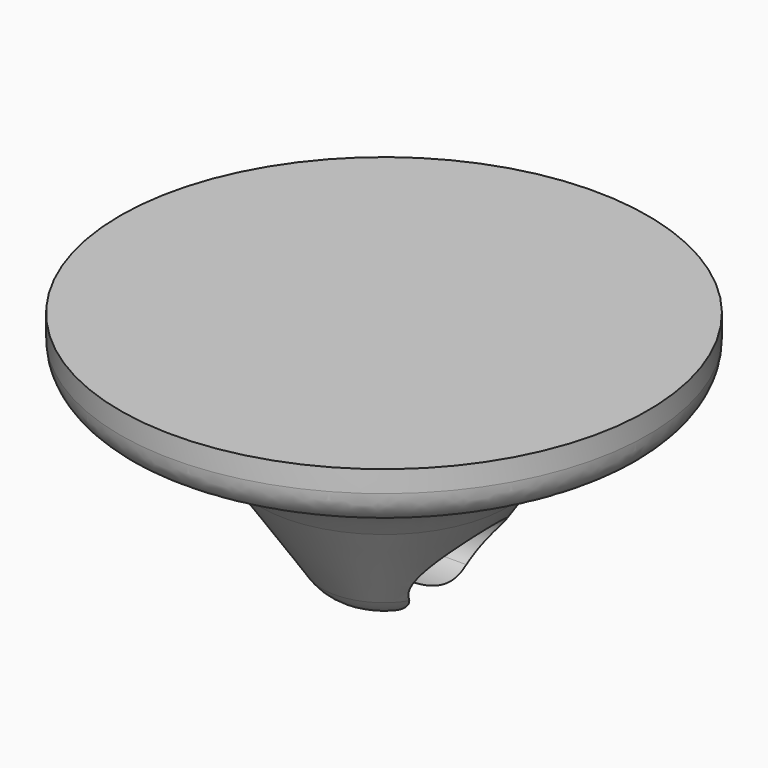
from build123d import *

# Parameters (mm, degrees)
F3_R          = 2
F4_R          = 3
F6_DEPTH      = 15.0010001
F6_DEPTH_BACK = 15.0010001
F7_T1_DEPTH   = 11.5921148274


# Not quite as in the source:
# - a fillet or chamfer that OpenCascade refuses, or shapes differently, is made with other operations: its cross-section is extruded or revolved along the edge and cut away or added
# - a feature of the source that left no trace in its solid (it failed there, or was rolled back) is left out


with BuildPart() as f1:
    # F0 (on Front) → F1 (revolve)
    with BuildSketch(Plane.XZ):
        Polygon((0, -13.9897428453), (0, 0), (-15, 0), (-15, -3), (-10, -3), (-2.61932757, -13.9897428453), align=None)
    revolve(axis=Axis((0, 0, -6.9948714226), (0, 0, 1)))

    # F2: fillet of radius 10 on 1 edges, made by hand

    # F2_s1 → F2_t2 (revolve)
    with BuildSketch(Plane.XZ):
        with BuildLine():
            ThreePointArc((-15, -3), (-10.4835294041, -4.2493813133), (-7.0321290602, -7.4191283024))
            Line((-7.0321290602, -7.4191283024), (-10, -3))
            Line((-10, -3), (-15, -3))
        make_face()
    revolve(axis=Axis((0, 0, -3), (0, 0, 1)))

    # F3
    f3_edges = [f1.edges().sort_by_distance(p)[0] for p in [
        (15, 0, -3),
    ]]
    fillet(f3_edges, radius=F3_R)

    # F4
    f4_edges = [f1.edges().sort_by_distance(p)[0] for p in [
        (2.619328, 0, -13.989743),
    ]]
    fillet(f4_edges, radius=F4_R)

    # F5 (on Right) → F6 (cut, two sides)
    with BuildSketch(Plane.YZ) as f6_sk:
        with BuildLine():
            Line((1.5, -14.6206104997), (1.5, -12.9897428453))
            ThreePointArc((1.5, -12.9897428453), (0, -8.4897428453), (-1.5, -12.9897428453))
            Line((-1.5, -12.9897428453), (-1.5, -14.6206104997))
            Line((-1.5, -14.6206104997), (1.5, -14.6206104997))
        make_face()
    extrude(amount=-F6_DEPTH, mode=Mode.SUBTRACT)
    extrude(f6_sk.sketch, amount=F6_DEPTH_BACK, mode=Mode.SUBTRACT)

    # F7: fillet of radius 3 on 2 edges, made by hand

    # F7_s2 → F7_t1 (cut)
    with BuildSketch(Plane.YZ.offset(-5.7960574137)):
        with BuildLine():
            ThreePointArc((-2.0454545455, -12.4271417817), (-1.6396122323, -13.2474864717), (-1.5, -14.1520205055))
            Line((-1.5, -14.1520205055), (-1.5, -12.9897428453))
            ThreePointArc((-1.5, -12.9897428453), (-1.7949072323, -12.7299462895), (-2.0454545455, -12.4271417817))
        make_face()
        with BuildLine():
            ThreePointArc((2.0454545455, -12.4271417817), (1.6396122323, -13.2474864717), (1.5, -14.1520205055))
            Line((1.5, -14.1520205055), (1.5, -12.9897428453))
            ThreePointArc((1.5, -12.9897428453), (1.7949072323, -12.7299462895), (2.0454545455, -12.4271417817))
        make_face()
    extrude(amount=F7_T1_DEPTH, mode=Mode.SUBTRACT)


solid = f1.part
